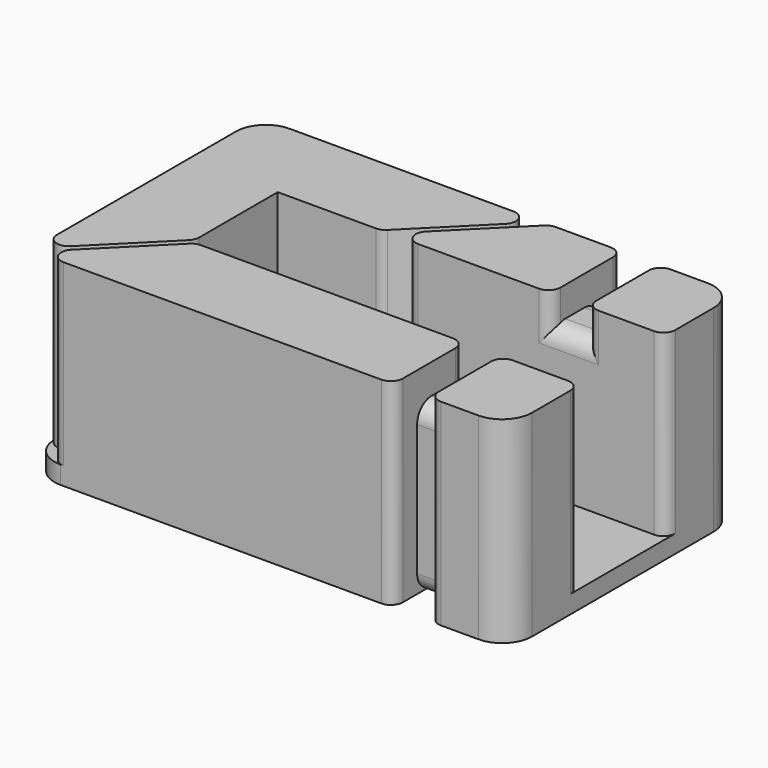
from build123d import *

# Parameters (mm, degrees)
F1_DEPTH = 3
F2_DEPTH = 30
F3_W     = 6
F3_H     = 5
F9_R     = 3
F10_R    = 2
F11_R    = 5


with BuildPart() as f1:
    # F0 (on Top) → F1 (new body)
    with BuildSketch(Plane.XY):
        Polygon((-63.0428932188, -24), (-48.0428932188, -9), (16.25, -9), (16.25, 9), (-30.0428932188, 9), (-15.0428932188, 24), (-16.4571067812, 24), (-31.4571067812, 9), (-48.75, 9), (-48.75, -8.2928932188), (-63.75, -23.2928932188), (-63.75, -24), align=None)
        Polygon((-63.75, 24), (-63.75, -23.2928932188), (-48.75, -8.2928932188), (-48.75, 9), (-31.4571067812, 9), (-16.4571067812, 24), align=None)
        Polygon((-30.0428932188, 9), (16.25, 9), (16.25, 24), (-15.0428932188, 24), align=None)
        Polygon((16.25, -9), (-48.0428932188, -9), (-63.0428932188, -24), (16.25, -24), align=None)
    extrude(amount=-F1_DEPTH)

    # F0 (on Top) → F2 (join)
    with BuildSketch(Plane.XY):
        Polygon((-63.75, 24), (-63.75, -23.2928932188), (-48.75, -8.2928932188), (-48.75, 9), (-31.4571067812, 9), (-16.4571067812, 24), align=None)
        Polygon((-30.0428932188, 9), (16.25, 9), (16.25, 24), (-15.0428932188, 24), align=None)
        Polygon((16.25, -9), (-48.0428932188, -9), (-63.0428932188, -24), (16.25, -24), align=None)
    extrude(amount=F2_DEPTH)

    # F7: sweep along a path in F6
    with BuildLine(Plane.YZ) as f7_path:
        Line((-24, -3), (-24, 30))
        Line((-24, 30), (-9, 30))
    # F3 (on face) → F7 (sweep, cut)
    with BuildSketch(Plane(origin=(0, 0, -3), x_dir=(1, 0, 0), z_dir=(0, 0, -1))):
        with Locations((0, 21.5)):
            Rectangle(F3_W, F3_H)
    sweep(path=f7_path.line, transition=Transition.RIGHT, mode=Mode.SUBTRACT)

    # F8: sweep along a path in F6
    with BuildLine(Plane.YZ) as f8_path:
        Line((24, -3), (24, 30))
        Line((24, 30), (9, 30))
    # F3 (on face) → F8 (sweep, cut)
    with BuildSketch(Plane(origin=(0, 0, -3), x_dir=(1, 0, 0), z_dir=(0, 0, -1))):
        with Locations((0, -21.5)):
            Rectangle(F3_W, F3_H)
    sweep(path=f8_path.line, transition=Transition.RIGHT, mode=Mode.SUBTRACT)

    # F9
    f9_edges = [f1.edges().sort_by_distance(p)[0] for p in [
        (0, -19, 25),
        (0, 19, 25),
        (0, -9, 25),
        (0, 9, 25),
        (0, -19, -3),
        (0, 19, -3),
    ]]
    fillet(f9_edges, radius=F9_R)

    # F10
    f10_edges = [f1.edges().sort_by_distance(p)[0] for p in [
        (-63.75, -23.292893, 15),
        (-63.042893, -24, 15),
        (-48.75, -8.292893, 15),
        (-48.042893, -9, 15),
        (-31.457107, 9, 15),
        (-30.042893, 9, 15),
        (-16.457107, 24, 15),
        (-15.042893, 24, 15),
        (16.25, 9, 15),
        (16.25, -9, 15),
        (-3, 9, 27.5),
        (3, 9, 27.5),
        (-3, -9, 27.5),
        (3, -9, 27.5),
        (-3, -24, 13.5),
        (-3, -9, 23.5),
        (3, -9, 23.5),
        (3, -24, 13.5),
        (-3, 24, 13.5),
        (-3, 9, 23.5),
        (3, 24, 13.5),
        (3, 9, 23.5),
    ]]
    fillet(f10_edges, radius=F10_R)

    # F11
    f11_edges = [f1.edges().sort_by_distance(p)[0] for p in [
        (16.25, -24, 13.5),
        (16.25, 24, 13.5),
        (-63.75, 24, 13.5),
        (-63.75, -24, -1.5),
    ]]
    fillet(f11_edges, radius=F11_R)


solid = f1.part
